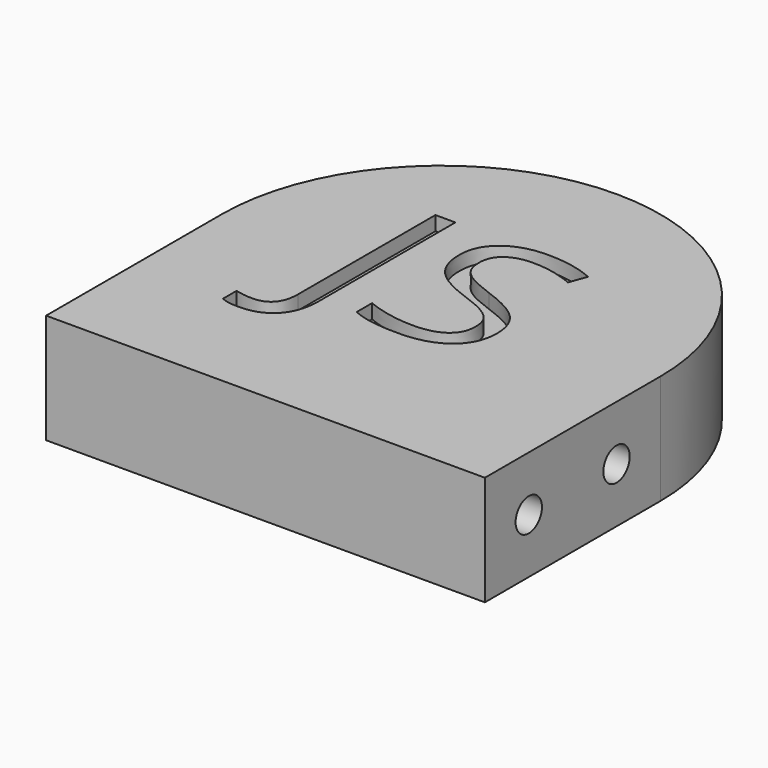
from build123d import *

# Parameters (mm, degrees)
F0_W         = 101.6
F0_H         = 50.8
F1_DEPTH     = 25.4
F2_R         = 3.81
F3_DEPTH     = 101.6
F4_TEXT_SIZE = 55.7667238422
F5_DEPTH     = 3.302


# Not quite as in the source:
# - Text() gives the source's letters only with a copy of the font that has no kerning and outlines rounded to 1/6400 em; it was checked with that copy


with BuildPart() as f1:
    # F0 (on Top) → F1 (new body)
    with BuildSketch(Plane.XY):
        with BuildLine():
            ThreePointArc((55.4109362923, 27.5538025672), (4.6109362923, 78.3538025672), (-46.1890637077, 27.5538025672))
            Line((-46.1890637077, 27.5538025672), (55.4109362923, 27.5538025672))
        make_face()
        with Locations((4.6109362923, 2.1538025672)):
            Rectangle(F0_W, F0_H)
    extrude(amount=-F1_DEPTH)

    # F2 (on face) → F3 (cut)
    with BuildSketch(Plane(origin=(-46.1890637077, 0, 0), x_dir=(0, -1, 0), z_dir=(-1, 0, 0))):
        with Locations((-14.8538025672, -12.7)):
            Circle(F2_R)
        with Locations((10.5461974328, -12.7)):
            Circle(F2_R)
    extrude(amount=-F3_DEPTH, mode=Mode.SUBTRACT)

    # F4 (on face) → F5 (cut)
    with BuildSketch(Plane.XY):
        with Locations((-21.0039680287, 11.6687277783)):
            Text('JS', F4_TEXT_SIZE, font='Open Sans', text_align=(TextAlign.LEFT, TextAlign.BOTTOM))
    extrude(amount=-F5_DEPTH, mode=Mode.SUBTRACT)


solid = f1.part
